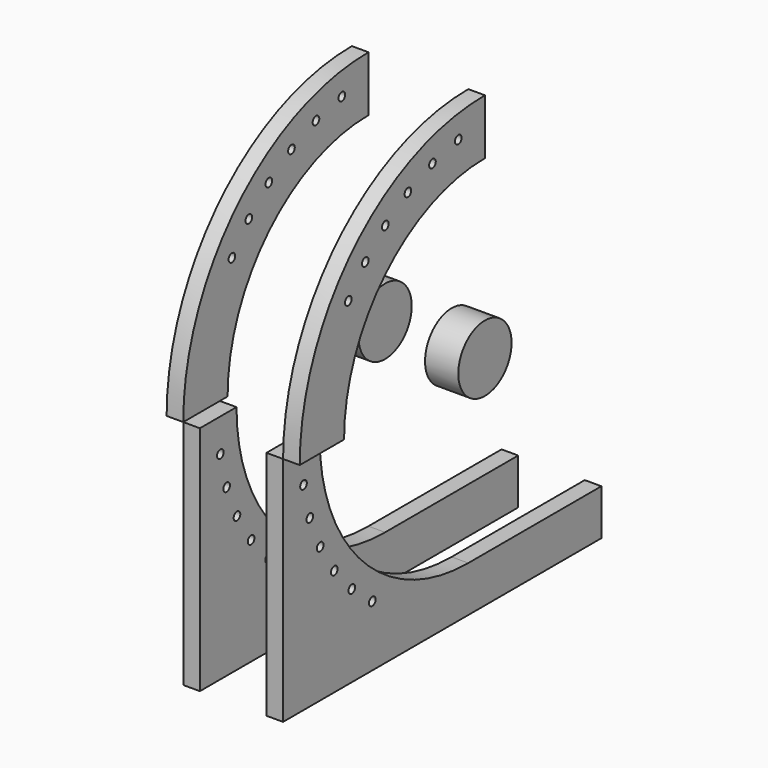
from build123d import *

# Parameters (mm, degrees)
F4_R      = 25.4
F5_DEPTH  = 25.4
F4_R_2    = 3.175
F4_W      = 127
F4_H      = 34.925
F6_DEPTH  = 12.7
F7_DEPTH  = 12.7
F9_R      = 3.175
F10_DEPTH = 12.7


# Not quite as in the source:
# - a variable given as a bare number and used for a length is read in inches; the dataset says mm whatever the document's units were


with BuildPart() as f5:
    # F4 (on offset) → F5 (new body)
    with BuildSketch(Plane.YZ.offset(25.4)):
        with Locations((0, 176.7078)):
            Circle(F4_R)
    extrude(amount=F5_DEPTH)


with BuildPart() as f6:
    # F4 (on offset) → F6 (new body)
    with BuildSketch(Plane.YZ.offset(25.4)):
        with BuildLine():
            ThreePointArc((-176.7078, 176.7078), (-124.9512836686, 51.7565163314), (0, 0))
            Line((0, 0), (0, 34.925))
            ThreePointArc((0, 34.925), (-100.2555793356, 76.4522206644), (-141.7828, 176.7078))
            Line((-141.7828, 176.7078), (-176.7078, 176.7078))
        make_face()
        with Locations((-91.5869799801, 46.4354289069)):
            Circle(F4_R_2, mode=Mode.SUBTRACT)
        with Locations((-111.1345130262, 62.6543669675)):
            Circle(F4_R_2, mode=Mode.SUBTRACT)
        with Locations((-127.8546728705, 81.7749384752)):
            Circle(F4_R_2, mode=Mode.SUBTRACT)
        with Locations((-141.3220819177, 103.3106969609)):
            Circle(F4_R_2, mode=Mode.SUBTRACT)
        with Locations((-151.1941158077, 126.713751182)):
            Circle(F4_R_2, mode=Mode.SUBTRACT)
        with Locations((-157.2196201212, 151.3887040243)):
            Circle(F4_R_2, mode=Mode.SUBTRACT)
        with Locations((63.5, 17.4625)):
            Rectangle(F4_W, F4_H)
    extrude(amount=F6_DEPTH)

    # F4 (on offset) → F7 (join)
    with BuildSketch(Plane.YZ.offset(25.4)):
        with BuildLine():
            Line((-176.7078, 0), (0, 0))
            ThreePointArc((0, 0), (-124.9512836686, 51.7565163314), (-176.7078, 176.7078))
            Line((-176.7078, 176.7078), (-176.7078, 0))
        make_face()
    extrude(amount=F7_DEPTH)


with BuildPart() as f10:
    # F9 (on offset) → F10 (new body)
    with BuildSketch(Plane.YZ.offset(38.1)):
        with BuildLine():
            ThreePointArc((-134.3914, 176.7078), (-95.0290702732, 271.7368702732), (0, 311.0992))
            Line((0, 311.0992), (0, 353.4156))
            ThreePointArc((0, 353.4156), (-124.9512836686, 301.6590836686), (-176.7078, 176.7078))
            Line((-176.7078, 176.7078), (-134.3914, 176.7078))
        make_face()
        with Locations((-130.3194857616, 268.2277279005)):
            Circle(F9_R, mode=Mode.SUBTRACT)
        with Locations((-114.1106092778, 287.7836048467)):
            Circle(F9_R, mode=Mode.SUBTRACT)
        with Locations((-94.9986447259, 304.5136021857)):
            Circle(F9_R, mode=Mode.SUBTRACT)
        with Locations((-73.4698196056, 317.992092047)):
            Circle(F9_R, mode=Mode.SUBTRACT)
        with Locations((-50.0718487676, 327.8761681631)):
            Circle(F9_R, mode=Mode.SUBTRACT)
        with Locations((-25.4, 333.9143697485)):
            Circle(F9_R, mode=Mode.SUBTRACT)
    extrude(amount=F10_DEPTH)


with BuildPart() as f11_1:
    # F11: instance of F10
    add(f10.part.mirror(Plane.YZ))


with BuildPart() as f11_2:
    # F11: instance of F5
    add(f5.part.mirror(Plane.YZ))


with BuildPart() as f11_3:
    # F11: instance of F6
    add(f6.part.mirror(Plane.YZ))


solid = Compound([f5.part, f6.part, f10.part, f11_1.part, f11_2.part, f11_3.part])
